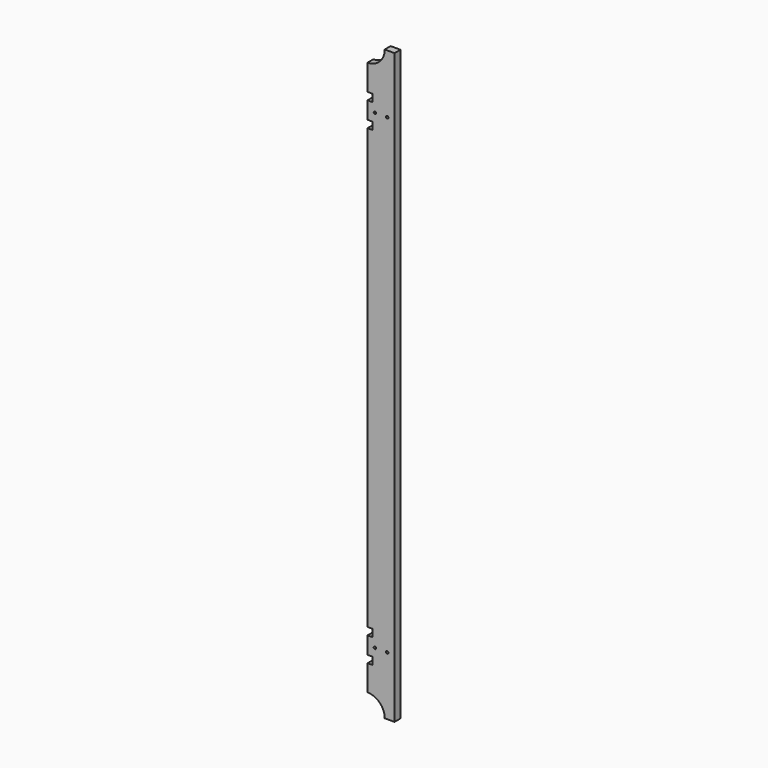
from build123d import *

# Parameters (mm, degrees)
F1_DEPTH = 38.1
F3_D     = 12.7
F4_W     = 25.4
F4_H     = 38.1
F5_DEPTH = 38.101


# Not quite as in the source:
# - a length typed as a fraction of an inch, garbled in the dataset ("3 / 203.2 mm" for 3/8 in), is restored


with BuildPart() as f1:
    # F0 (on Front) → F1 (new body)
    with BuildSketch(Plane.XZ):
        with BuildLine():
            ThreePointArc((88.9, 0), (62.8617928475, -62.8617928475), (0, -88.9))
            Line((0, -88.9), (0, -2959.1))
            ThreePointArc((0, -2959.1), (62.8617928475, -2985.1382071525), (88.9, -3048))
            Line((88.9, -3048), (139.7, -3048))
            Line((139.7, -3048), (139.7, 0))
            Line((139.7, 0), (88.9, 0))
        make_face()
    extrude(amount=F1_DEPTH)

    # F3 (through all)
    with Locations(Plane.XZ.offset(38.1)):
        with Locations((38.1, -2743.2), (101.6, -2743.2), (38.1, -304.8), (101.6, -304.8)):
            Hole(F3_D / 2)

    # F4 (on face) → F5 (cut, through all)
    with BuildSketch(Plane.XZ.offset(38.1)):
        with Locations((12.7, -241.3)):
            Rectangle(F4_W, F4_H)
        with Locations((12.7, -368.3)):
            Rectangle(F4_W, F4_H)
        with Locations((12.7, -2679.7)):
            Rectangle(F4_W, F4_H)
        with Locations((12.7, -2806.7)):
            Rectangle(F4_W, F4_H)
    extrude(amount=-F5_DEPTH, mode=Mode.SUBTRACT)


solid = f1.part
